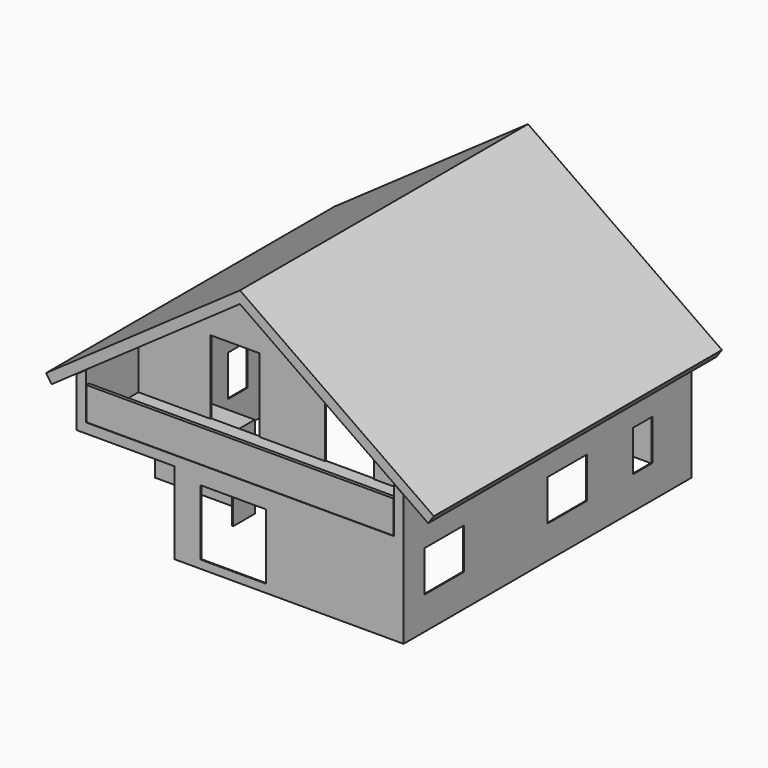
from build123d import *

# Parameters (mm, degrees)
F1_DEPTH      = 5500
F1_DEPTH_BACK = 5500
F2_W          = 3000
F2_H          = 2500
F3_DEPTH      = 2000
F5_DEPTH      = 5500
F5_DEPTH_BACK = 5500
F6_W          = 3000
F6_H          = 2500
F7_DEPTH      = 1000
F8_T          = -30
F9_W          = 1500
F9_H          = 2250
F10_DEPTH     = 30
F11_W         = 1400
F11_H         = 2250
F12_DEPTH     = 30
F13_W         = 2000
F13_H         = 2000
F14_DEPTH     = 30
F15_W         = 1500
F15_H         = 1250
F15_W_2       = 750
F16_DEPTH     = 30
F17_W         = 9380
F17_H         = 1000
F18_DEPTH     = 100
F19_W         = 750
F19_H         = 1250
F20_DEPTH     = 30
F21_W         = 750
F21_H         = 1250
F21_W_2       = 1000
F21_H_2       = 2250
F22_DEPTH     = 30
F23_W         = 750
F23_H         = 1250
F24_DEPTH     = 30


# Not quite as in the source:
# - a feature names something its author has since deleted; it is built from what else it names


with BuildPart() as f1:
    # F0 (on Front) → F1 (new body, two sides)
    with BuildSketch(Plane.XZ) as f1_sk:
        Polygon((-5000, 4000), (-5000, 0), (5000, 0), (5000, 4000), (0, 7501.0376910485), align=None)
    extrude(amount=F1_DEPTH)
    extrude(f1_sk.sketch, amount=-F1_DEPTH_BACK)

    # F2 (on face) → F3 (cut)
    with BuildSketch(Plane.XZ.offset(5500)):
        Polygon((4700, 4210.0622614629), (0, 7501.0376910485), (-4700, 4210.0622614629), (-4700, 2800), (4700, 2800), align=None)
        with Locations((-3500, 1250)):
            Rectangle(F2_W, F2_H)
    extrude(amount=-F3_DEPTH, mode=Mode.SUBTRACT)

    # F6 (on face) → F7 (cut)
    with BuildSketch(Plane.XZ.offset(3500)):
        with Locations((-3500, 1250)):
            Rectangle(F6_W, F6_H)
    extrude(amount=-F7_DEPTH, mode=Mode.SUBTRACT)

    # F8
    f8_openings = [f1.faces().sort_by_distance(p)[0] for p in [
        (311.881188, 356.435644, 0),
    ]]
    offset(amount=F8_T, openings=f8_openings, kind=Kind.INTERSECTION)

    # F9 (on face) → F10 (cut, through all)
    with BuildSketch(Plane.XZ.offset(3500)):
        with Locations((-1750, 3925)):
            Rectangle(F9_W, F9_H)
        with Locations((1750, 3925)):
            Rectangle(F9_W, F9_H)
    extrude(amount=-F10_DEPTH, mode=Mode.SUBTRACT)

    # F11 (on face) → F12 (cut, through all)
    with BuildSketch(Plane(origin=(-2000, 0, 0), x_dir=(0, -1, 0), z_dir=(-1, 0, 0))):
        with Locations((4000, 1125)):
            Rectangle(F11_W, F11_H)
    extrude(amount=-F12_DEPTH, mode=Mode.SUBTRACT)

    # F13 (on face) → F14 (cut, through all)
    with BuildSketch(Plane.XZ.offset(5500)):
        with Locations((-200, 1250)):
            Rectangle(F13_W, F13_H)
    extrude(amount=-F14_DEPTH, mode=Mode.SUBTRACT)

    # F15 (on face) → F16 (cut, through all)
    with BuildSketch(Plane.YZ.offset(5000)):
        with Locations((-3950, 1625)):
            Rectangle(F15_W, F15_H)
        with Locations((750, 1625)):
            Rectangle(F15_W, F15_H)
        with Locations((3625, 1625)):
            Rectangle(F15_W_2, F15_H)
    extrude(amount=-F16_DEPTH, mode=Mode.SUBTRACT)

    # F19 (on face) → F20 (cut, through all)
    with BuildSketch(Plane.XZ.offset(2500)):
        with Locations((-3500, 1625)):
            Rectangle(F19_W, F19_H)
    extrude(amount=-F20_DEPTH, mode=Mode.SUBTRACT)

    # F21 (on face) → F22 (cut, through all)
    with BuildSketch(Plane(origin=(0, 5500, 0), x_dir=(-1, 0, 0), z_dir=(0, 1, 0))):
        with Locations((-2625, 1625)):
            Rectangle(F21_W, F21_H)
        with Locations((-625, 1625)):
            Rectangle(F21_W, F21_H)
        with Locations((700, 1125)):
            Rectangle(F21_W_2, F21_H_2)
        with Locations((-2625, 4425)):
            Rectangle(F21_W, F21_H)
        with Locations((-625, 4425)):
            Rectangle(F21_W, F21_H)
        with Locations((2875, 4425)):
            Rectangle(F21_W, F21_H)
    extrude(amount=-F22_DEPTH, mode=Mode.SUBTRACT)

    # F23 (on face) → F24 (cut, through all)
    with BuildSketch(Plane(origin=(-5000, 0, 0), x_dir=(0, -1, 0), z_dir=(-1, 0, 0))):
        with Locations((-3625, 1625)):
            Rectangle(F23_W, F23_H)
        with Locations((-625, 1625)):
            Rectangle(F23_W, F23_H)
    extrude(amount=-F24_DEPTH, mode=Mode.SUBTRACT)


with BuildPart() as f5:
    # F4 (on Front) → F5 (new body, two sides)
    with BuildSketch(Plane.XZ) as f5_sk:
        Polygon((-5922.0729309053, 3732.797705517), (-5750, 3487.0520922303), (0, 7513.2454369362), (5750, 3487.0520922303), (5922.0729309053, 3732.797705517), (0, 7879.4778135646), align=None)
    extrude(amount=F5_DEPTH)
    extrude(f5_sk.sketch, amount=-F5_DEPTH_BACK)


with BuildPart() as f18:
    # F17 (on face) → F18 (new body)
    with BuildSketch(Plane.XZ.offset(5500)):
        with Locations((0, 3310)):
            Rectangle(F17_W, F17_H)
    extrude(amount=-F18_DEPTH)


solid = Compound([f1.part, f5.part, f18.part])
